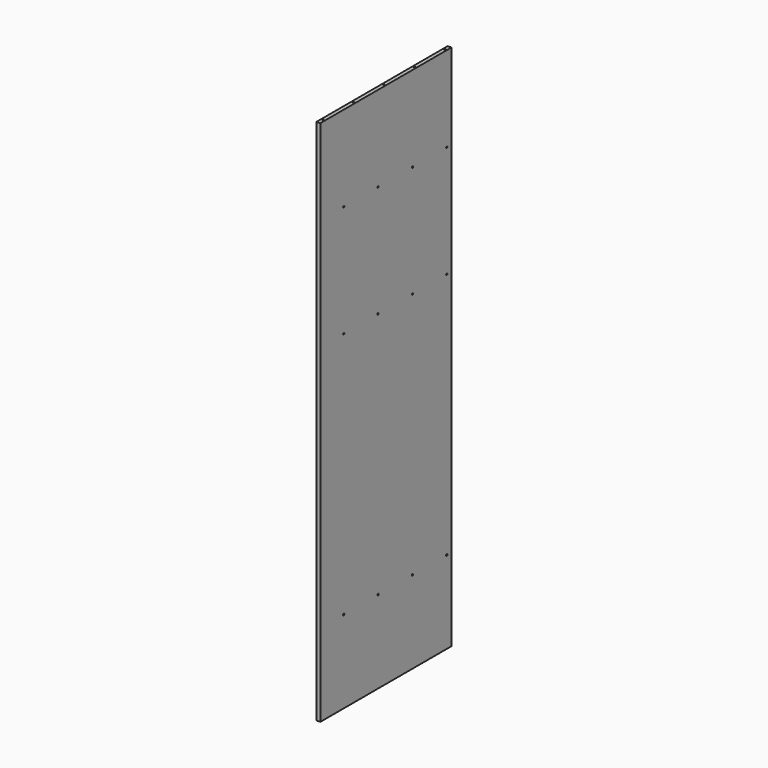
from build123d import *

# Parameters (mm, degrees)
F0_W           = 700
F0_H           = 2250
F1_DEPTH       = 8
F3_D           = 5
F3_DEPTH       = 35
F3_CSINK_D     = 7
F3_CSINK_ANGLE = 90
F3_TIP         = 1.5021515476
F5_D           = 7


# Not quite as in the source:
# - a feature names something its author has since deleted; it is built from what else it names


with BuildPart() as f1:
    # F0 (on Right) → F1 (new body, symmetric)
    with BuildSketch(Plane.YZ):
        Rectangle(F0_W, F0_H)
    extrude(amount=F1_DEPTH, both=True)

    # F3
    with Locations(Plane.XY.offset(1125)):
        with Locations((0, 325), (0, 162.5), (0, 0), (0, -162.5), (0, -325)):
            CounterSinkHole(F3_D / 2, F3_CSINK_D / 2, depth=F3_DEPTH, counter_sink_angle=F3_CSINK_ANGLE)
            with Locations((0, 0, -(F3_DEPTH + F3_TIP / 2))):  # 118° drill point
                Cone(0, F3_D / 2, F3_TIP, mode=Mode.SUBTRACT)

    # F5 (through all)
    with Locations(Plane.YZ.offset(8)):
        with Locations((-225, 760), (-42, 760), (142, 760), (325, 760), (325, 283), (142, 283), (-42, 283), (-225, 283), (325, -772), (142, -772), (-42, -772), (-225, -772)):
            Hole(F5_D / 2)


solid = f1.part
